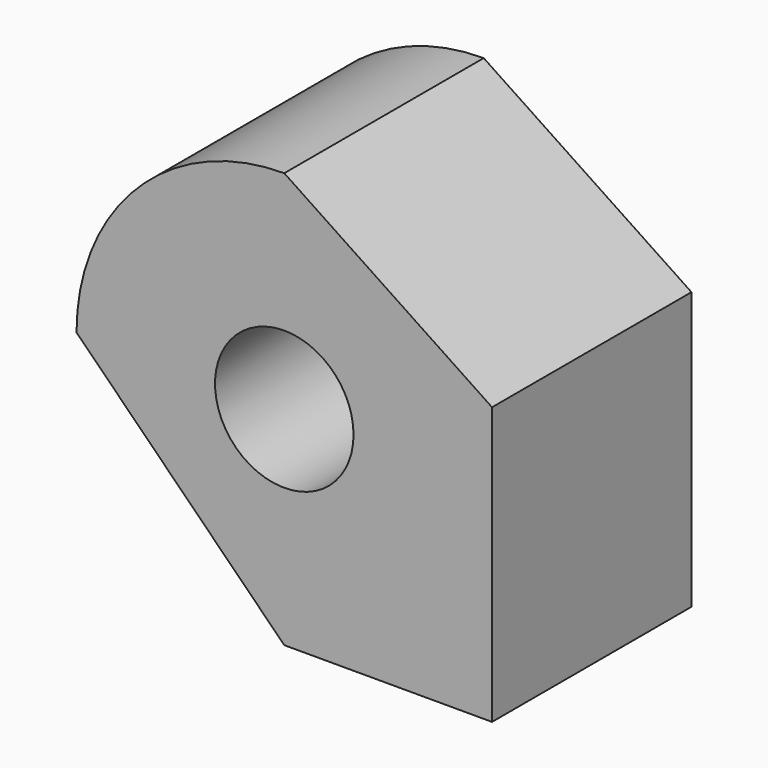
from build123d import *

# Parameters (mm, degrees)
F0_R     = 5
F1_DEPTH = 9
F2_R     = 14.99999


# Not quite as in the source:
# - a fillet or chamfer is up to 0.001 mm smaller than in the source, because OpenCascade refuses the exact size


with BuildPart() as f1:
    # F0 (on Front) → F1 (new body, symmetric)
    with BuildSketch(Plane.XZ):
        Polygon((0, 15), (15, 0), (30, 0), (30, 20), (15, 30), (0, 30), align=None)
        with Locations((15, 15)):
            Circle(F0_R, mode=Mode.SUBTRACT)
    extrude(amount=F1_DEPTH, both=True)

    # F2 (radius 15 in the source; OpenCascade refuses exactly that, so slightly less here)
    f2_edges = [f1.edges().sort_by_distance(p)[0] for p in [
        (0, 0, 30),
    ]]
    fillet(f2_edges, radius=F2_R)


solid = f1.part
